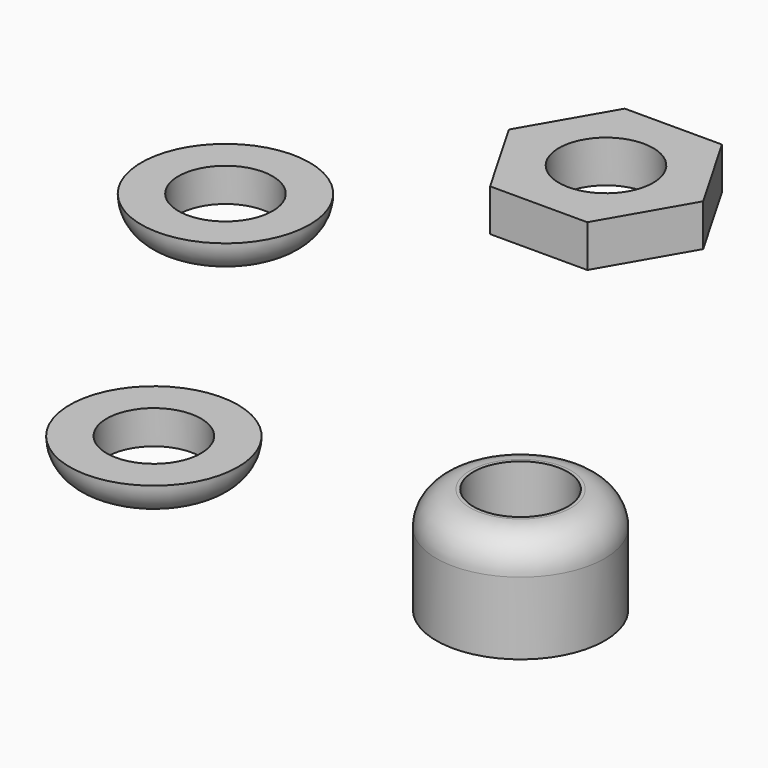
from build123d import *

# Parameters (mm, degrees)
F0_R      = 6.35
F1_DEPTH  = 2.54
F2_R      = 2.53999
F2_2_R    = 2.53999
F3_R      = 3.556
F4_DEPTH  = 2.54
F5_R      = 3.556
F6_DEPTH  = 2.54
F7_R      = 6.35
F8_DEPTH  = 8.001
F9_R      = 2.54
F11_R     = 3.556
F12_DEPTH = 11.1506
F14_DEPTH = 3.175
F15_R     = 3.556
F16_DEPTH = 3.175


# Not quite as in the source:
# - a fillet or chamfer is up to 0.001 mm smaller than in the source, because OpenCascade refuses the exact size
# - a feature names something its author has since deleted; it is built from what else it names


with BuildPart() as f1:
    # F0 (on Top) → F1 (new body)
    with BuildSketch(Plane.XY):
        Circle(F0_R)
    extrude(amount=F1_DEPTH)

    # F2 (radius 2.54 in the source; OpenCascade refuses exactly that, so slightly less here)
    f2_edges = [f1.edges().sort_by_distance(p)[0] for p in [
        (-6.35, 0, 0),
    ]]
    fillet(f2_edges, radius=F2_R)

    # F3 (on face) → F4 (cut)
    with BuildSketch(Plane(origin=(0, 0, 0), x_dir=(1, 0, 0), z_dir=(0, 0, -1))):
        Circle(F3_R)
    extrude(amount=-F4_DEPTH, mode=Mode.SUBTRACT)


with BuildPart() as f1b:
    # F0 (on Top) → F1, piece 2 (new body)
    with BuildSketch(Plane.XY):
        with Locations((-16.0212460905, 26.7825610936)):
            Circle(F0_R)
    extrude(amount=F1_DEPTH)

    # F2#2 (radius 2.54 in the source; OpenCascade refuses exactly that, so slightly less here)
    f2_2_edges = [f1b.edges().sort_by_distance(p)[0] for p in [
        (-22.371246, 26.782561, 0),
    ]]
    fillet(f2_2_edges, radius=F2_2_R)

    # F5 (on face) → F6 (cut)
    with BuildSketch(Plane(origin=(0, 0, 0), x_dir=(1, 0, 0), z_dir=(0, 0, -1))):
        with Locations((-16.0212460905, -26.7825610936)):
            Circle(F5_R)
    extrude(amount=-F6_DEPTH, mode=Mode.SUBTRACT)


with BuildPart() as f8:
    # F7 (on Top) → F8 (new body)
    with BuildSketch(Plane.XY):
        with Locations((27.6708697799, 0)):
            Circle(F7_R)
    extrude(amount=F8_DEPTH)

    # F9
    f9_edges = [f8.edges().sort_by_distance(p)[0] for p in [
        (21.32087, 0, 8.001),
    ]]
    fillet(f9_edges, radius=F9_R)

    # F11 (on face) → F12 (cut)
    with BuildSketch(Plane.XY.offset(8.001)):
        with Locations((27.6708697799, 0)):
            Circle(F11_R)
    extrude(amount=-F12_DEPTH, mode=Mode.SUBTRACT)


with BuildPart() as f14:
    # F13 (on Top) → F14 (new body)
    with BuildSketch(Plane.XY):
        Polygon((-3.6661742094, 36.2963240518), (3.6661742094, 36.2963240518), (7.3323484187, 42.6463240518), (3.6661742094, 48.9963240518), (-3.6661742094, 48.9963240518), (-7.3323484187, 42.6463240518), align=None)
    extrude(amount=F14_DEPTH)

    # F15 (on face) → F16 (cut)
    with BuildSketch(Plane.XY.offset(3.175)):
        with Locations((0, 42.6463240518)):
            Circle(F15_R)
    extrude(amount=-F16_DEPTH, mode=Mode.SUBTRACT)


solid = Compound([f1.part, f1b.part, f8.part, f14.part])
